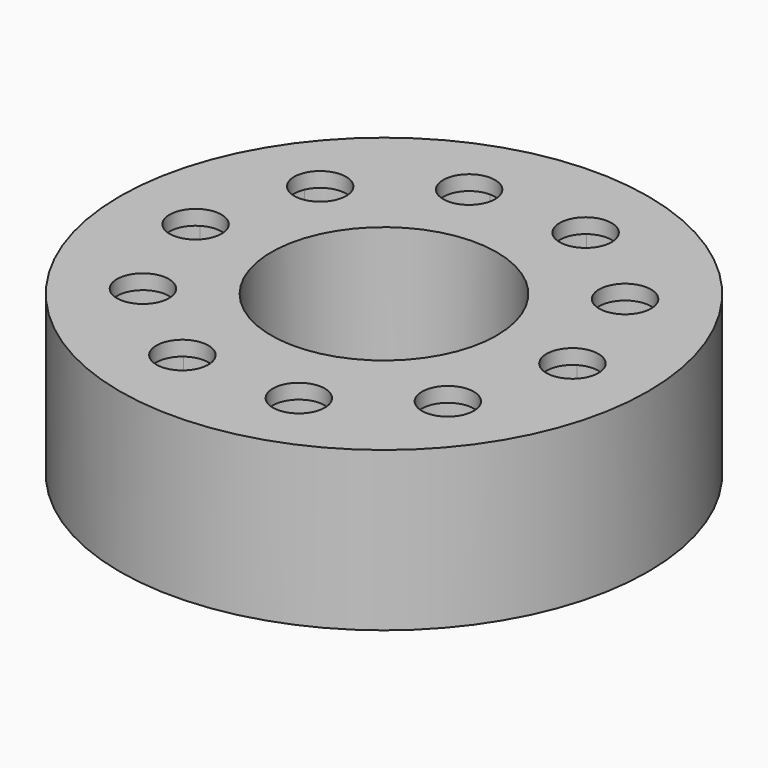
from build123d import *

# Parameters (mm, degrees)
F0_R            = 17.8
F0_R_2          = 7.6
F0_R_3          = 1.75
F1_DEPTH        = 10.7
F2_DEPTH        = 9.7
F2_COPIES_COUNT = 10
F3_DEPTH        = 10.7
F3_COPIES_COUNT = 10


# Not quite as in the source:
# - a pattern or mirror of a feature is missing from the dataset's text; its kind, count and spacing are read off the source's solid


with BuildPart() as f1:
    # F0 (on Top) → F1 (new body)
    with BuildSketch(Plane.XY):
        Circle(F0_R)
        Circle(F0_R_2, mode=Mode.SUBTRACT)
        with BuildLine():
            ThreePointArc((14.45, 2.5588083164), (15.4418059742, 1.4465476141), (15.8, 0))
            ThreePointArc((15.8, 0), (15.4418059742, -1.4465476141), (14.45, -2.5588083164))
            Line((14.45, -2.5588083164), (14.45, -3.5))
            Line((14.45, -3.5), (10.95, -3.5))
            Line((10.95, -3.5), (10.95, -2.5588083164))
            ThreePointArc((10.95, -2.5588083164), (9.6, 0), (10.95, 2.5588083164))
            Line((10.95, 2.5588083164), (10.95, 3.5))
            Line((10.95, 3.5), (14.45, 3.5))
            Line((14.45, 3.5), (14.45, 2.5588083164))
        make_face(mode=Mode.SUBTRACT)
        with BuildLine():
            ThreePointArc((14.45, -2.5588083164), (15.4418059742, -1.4465476141), (15.8, 0))
            ThreePointArc((15.8, 0), (15.4418059742, 1.4465476141), (14.45, 2.5588083164))
            ThreePointArc((14.45, 2.5588083164), (12.7, 3.1), (10.95, 2.5588083164))
            ThreePointArc((10.95, 2.5588083164), (9.6, 0), (10.95, -2.5588083164))
            ThreePointArc((10.95, -2.5588083164), (12.7, -3.1), (14.45, -2.5588083164))
        make_face()
        with Locations((12.7, 0)):
            Circle(F0_R_3, mode=Mode.SUBTRACT)
        with Locations((12.7, 0)):
            Circle(F0_R_3)
        with BuildLine():
            Line((14.45, -3.5), (14.45, -2.5588083164))
            ThreePointArc((14.45, -2.5588083164), (12.7, -3.1), (10.95, -2.5588083164))
            Line((10.95, -2.5588083164), (10.95, -3.5))
            Line((10.95, -3.5), (14.45, -3.5))
        make_face()
        with BuildLine():
            ThreePointArc((10.95, 2.5588083164), (12.7, 3.1), (14.45, 2.5588083164))
            Line((14.45, 2.5588083164), (14.45, 3.5))
            Line((14.45, 3.5), (10.95, 3.5))
            Line((10.95, 3.5), (10.95, 2.5588083164))
        make_face()
    extrude(amount=F1_DEPTH)

    # F0 (on Top) → F2 (cut)
    with BuildSketch(Plane.XY):
        with BuildLine():
            ThreePointArc((14.45, -2.5588083164), (15.4418059742, -1.4465476141), (15.8, 0))
            ThreePointArc((15.8, 0), (15.4418059742, 1.4465476141), (14.45, 2.5588083164))
            ThreePointArc((14.45, 2.5588083164), (12.7, 3.1), (10.95, 2.5588083164))
            ThreePointArc((10.95, 2.5588083164), (9.6, 0), (10.95, -2.5588083164))
            ThreePointArc((10.95, -2.5588083164), (12.7, -3.1), (14.45, -2.5588083164))
        make_face()
        with Locations((12.7, 0)):
            Circle(F0_R_3, mode=Mode.SUBTRACT)
        with Locations((12.7, 0)):
            Circle(F0_R_3)
    f2 = extrude(amount=F2_DEPTH, mode=Mode.SUBTRACT)

    # F2_copies: F2 ×10 about axis
    f2_copies_axis = Axis((0, 0, 0), (0, 0, 1))
    for i in range(1, F2_COPIES_COUNT):
        add(f2.rotate(f2_copies_axis, i * 360 / F2_COPIES_COUNT), mode=Mode.SUBTRACT)

    # F0 (on Top) → F3 (cut, through all)
    with BuildSketch(Plane.XY):
        with Locations((12.7, 0)):
            Circle(F0_R_3)
    f3 = extrude(amount=F3_DEPTH, mode=Mode.SUBTRACT)

    # F3_copies: F3 ×10 about axis
    f3_copies_axis = Axis((0, 0, 0), (0, 0, 1))
    for i in range(1, F3_COPIES_COUNT):
        add(f3.rotate(f3_copies_axis, i * 360 / F3_COPIES_COUNT), mode=Mode.SUBTRACT)


solid = f1.part
